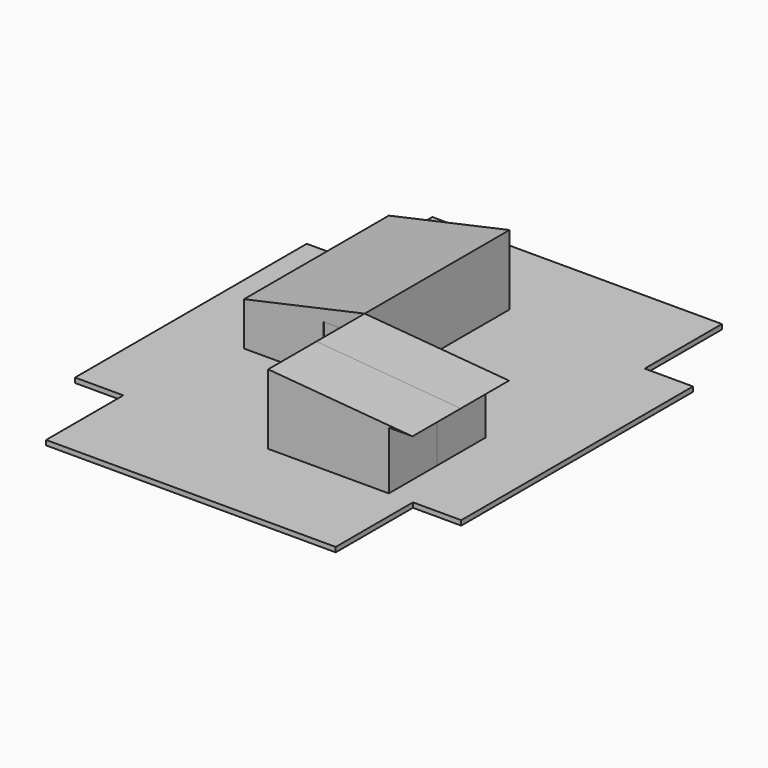
from build123d import *

# Parameters (mm, degrees)
F2_W      = 5000
F2_H      = 2400
F3_DEPTH  = 2500
F4_DEPTH  = 2500
F5_DEPTH  = 7500
F6_W      = 12000
F6_H      = 4000
F7_DEPTH  = 200
F8_W      = 700
F8_H      = 600
F9_DEPTH  = 100
F10_W     = 700
F10_H     = 1350
F11_DEPTH = 25


# Not quite as in the source:
# - a feature names something its author has since deleted; it is built from what else it names


with BuildPart() as f3:
    # F2 (on offset) → F3 (new body)
    with BuildSketch(Plane.XZ.offset(13000)):
        with Locations((2500, 1200)):
            Rectangle(F2_W, F2_H)
        Polygon((0, 2900), (0, 2400), (5000, 2400), (5979.1303715507, 2400), align=None)
    extrude(amount=F3_DEPTH)


with BuildPart() as f4:
    # F4 (new): a face of the model
    f4_faces = [f3.part.faces().sort_by_distance(p)[0] for p in [
        (2500, -15500, 66.4529909033),
    ]]
    extrude(f4_faces, amount=F4_DEPTH)


with BuildPart() as f5:
    # F2 (on offset) → F5 (new body)
    with BuildSketch(Plane.XZ.offset(13000)):
        Polygon((-5000, 0), (0, 0), (0, 2400), (0, 2900), (-5000, 1800), align=None)
    extrude(amount=-F5_DEPTH)

    # F8 (on face) → F9 (cut)
    with BuildSketch(Plane(origin=(-5000, 0, 0), x_dir=(0, -1, 0), z_dir=(-1, 0, 0))):
        with Locations((11400, 1000)):
            Rectangle(F8_W, F8_H)
        with Locations((12100, 1000)):
            Rectangle(F8_W, F8_H)
    extrude(amount=-F9_DEPTH, mode=Mode.SUBTRACT)

    # F10 (on face) → F11 (cut)
    with BuildSketch(Plane.XZ.offset(13000)):
        with Locations((-1350, 1375)):
            Rectangle(F10_W, F10_H)
        with Locations((-650, 1375)):
            Rectangle(F10_W, F10_H)
    extrude(amount=-F11_DEPTH, mode=Mode.SUBTRACT)


with BuildPart() as f7:
    # F6 (on Top) → F7 (new body)
    with BuildSketch(Plane.XY):
        with Locations((0, -20000)):
            Rectangle(F6_W, F6_H)
        Polygon((-6000, -6000), (-8000, -6000), (-8000, -18000), (-6000, -18000), (6000, -18000), (8000, -18000), (8000, -6000), (6000, -6000), align=None)
        with Locations((0, -4000)):
            Rectangle(F6_W, F6_H)
    extrude(amount=-F7_DEPTH)


solid = Compound([f3.part, f4.part, f5.part, f7.part])
